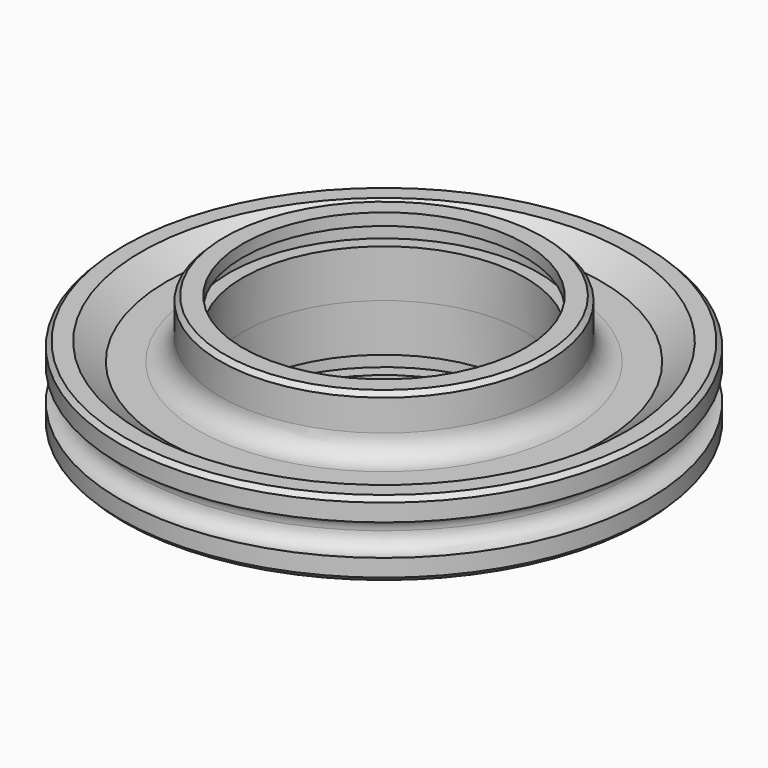
from build123d import *
from build123d import SkipClean  # not in build123d's __all__

# Parameters (mm, degrees)
F2_R    = 0.889
F4_SIZE = 0.254
F5_R    = 1.27


with BuildPart() as f1:
    # F0 (on Front) → F1 (revolve)
    with BuildSketch(Plane.XZ):
        Polygon((8.0391, 2.7178), (8.0391, 0), (15.0368, 0), (15.0368, 2.1336), (13.8207983748, 2.1336), (12.3698, 1.1176), (9.3218, 1.1176), (9.3218, 4.4196), (8.0391, 4.4196), (8.0391, 3.7338), (8.8011, 3.7338), (8.8011, 2.7178), align=None)
    revolve(axis=Axis((0, 0, 18.0261821733), (0, 0, 1)))

    # F2 (on Front) → F3 (revolve, cut)
    with BuildSketch(Plane.XZ):
        with Locations((15.0368, 0)):
            Circle(F2_R)
    revolve(axis=Axis((0, 0, 18.0261821733), (0, 0, 1)), mode=Mode.SUBTRACT)

    # F4
    f4_edges = [f1.edges().sort_by_distance(p)[0] for p in [
        (-15.0368, 0, 2.1336),
        (-9.3218, 0, 4.4196),
    ]]
    chamfer(f4_edges, length=F4_SIZE)

    # F5
    f5_edges = [f1.edges().sort_by_distance(p)[0] for p in [
        (-9.3218, 0, 1.1176),
    ]]
    fillet(f5_edges, radius=F5_R)

    # F6: F1 across plane


with BuildPart() as f1_1:
    add(f1.part, clean=False)
    with SkipClean():  # cleaning this boolean's faces spoils the solid; the shape is the same uncleaned
        add(f1.part.mirror(Plane.XY), clean=False)


solid = f1_1.part
